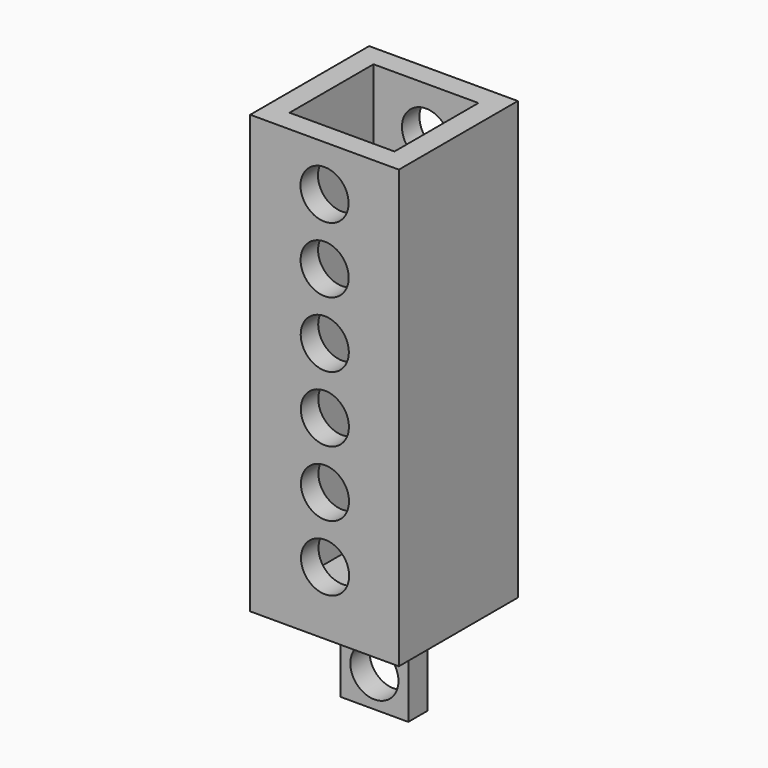
from build123d import *

# Parameters (mm, degrees)
F0_W        = 15.5
F0_H        = 5.5
F1_DEPTH    = 20
F2_R        = 5.5
F3_DEPTH    = 5.5
F4_W        = 34
F4_H        = 34
F4_W_2      = 15.5
F4_H_2      = 5.5
F5_DEPTH    = 100
F6_T        = 5
F6_T3_DEPTH = 15.5
F6_T5_DEPTH = 25.5
F7_R        = 5.5
F8_DEPTH    = 34


# Not quite as in the source:
# - a shell that OpenCascade refuses in one call is made with other operations: the cavity is built on its own and cut out


with BuildPart() as f1:
    # F0 (on Top) → F1 (new body)
    with BuildSketch(Plane.XY):
        Rectangle(F0_W, F0_H)
    extrude(amount=F1_DEPTH)

    # F2 (on face) → F3 (cut, through all)
    with BuildSketch(Plane.XZ.offset(2.75)):
        with Locations((0, 7.5)):
            Circle(F2_R)
    extrude(amount=-F3_DEPTH, mode=Mode.SUBTRACT)

    # F4 (on face) → F5 (join)
    with BuildSketch(Plane.XY.offset(20)):
        Rectangle(F4_W, F4_H)
        Rectangle(F4_W_2, F4_H_2, mode=Mode.SUBTRACT)
        Rectangle(F4_W_2, F4_H_2)
    extrude(amount=F5_DEPTH)

    # F6: shell of thickness 5, made by hand


with BuildPart() as f6_core1:
    # F6_t2: copy of F1
    add(f1.part)

    # the walls: a layer under each face that stays
    f6_faces = [f6_core1.faces().sort_by_distance(p)[0] for p in [
        (17, 0, 70),
        (0, -17, 70),
        (0, 17, 70),
        (-11.3333333333, -11.3333333333, 20),
        (-17, 0, 70),
        (7.75, 0, 10),
        (5.1666666667, 2.75, 16.6666666667),
        (-7.75, 0, 10),
        (-5.1666666667, -2.75, 16.6666666667),
        (0, 0, 0),
        (-5.5, 0, 7.5),
    ]]
    thicken(f6_faces, amount=-F6_T, mode=Mode.SUBTRACT)

    # F6_s4 → F6_t3 (cut)
    with BuildSketch(Plane.XZ.offset(-7.75)):
        Polygon((7.8, 19.95), (7.75, 25), (2.75, 25), (2.75, 20), align=None)
        Polygon((-7.8, 19.95), (-7.75, 25), (-2.75, 25), (-2.75, 20), align=None)
    extrude(amount=F6_T3_DEPTH, mode=Mode.SUBTRACT)

    # F6_s6 → F6_t5 (cut)
    with BuildSketch(Plane.YZ.offset(-12.75)):
        Polygon((2.8, 19.95), (2.75, 25), (-2.25, 25), (-2.25, 20), align=None)
        Polygon((-2.8, 19.95), (-2.75, 25), (2.25, 25), (2.25, 20), align=None)
    extrude(amount=F6_T5_DEPTH, mode=Mode.SUBTRACT)


with BuildPart() as f1_1:
    add(f1.part)

    # what is left inside the walls is the cavity
    f6_cavity = [f6_core1.part.solids().sort_by_distance(p)[0] for p in [
        (11.95, 0, 88.333333),
    ]]
    add(f6_cavity, mode=Mode.SUBTRACT)

    # F7 (on face) → F8 (cut, through all)
    with BuildSketch(Plane(origin=(0, 17, 0), x_dir=(-1, 0, 0), z_dir=(0, 1, 0))):
        with Locations((0, 109.5)):
            Circle(F7_R)
        with Locations((-0.0251045674, 94.500021008)):
            Circle(F7_R)
        with Locations((-0.0502091347, 79.500042016)):
            Circle(F7_R)
        with Locations((-0.0753137021, 64.500063024)):
            Circle(F7_R)
        with Locations((-0.1004182694, 49.500084032)):
            Circle(F7_R)
        with Locations((-0.1255228368, 34.50010504)):
            Circle(F7_R)
    extrude(amount=-F8_DEPTH, mode=Mode.SUBTRACT)


solid = f1_1.part
